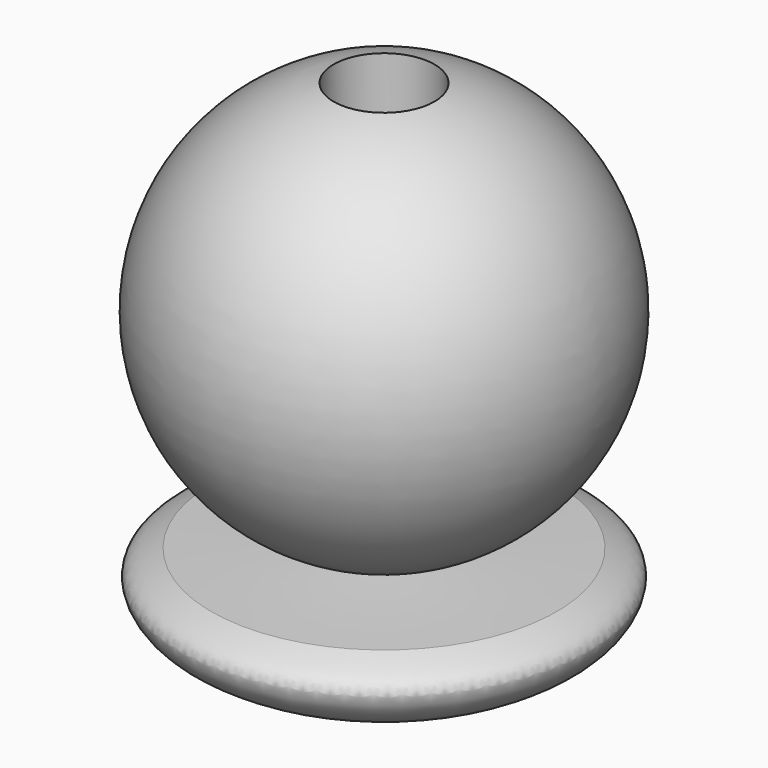
from build123d import *


with BuildPart() as f1:
    # F0 (on Front) → F1 (revolve)
    with BuildSketch(Plane.XZ):
        with BuildLine():
            Line((0, -57.654262), (0, -58.470906))
            ThreePointArc((0, -58.470906), (24.864604, -36.49857), (6.118411, -9.11952))
            Line((6.118411, -9.11952), (6.118411, -19.531853))
            Line((6.118411, -19.531853), (0, -19.531853))
            Line((0, -19.531853), (0, -57.654262))
        make_face()
        with BuildLine():
            add(Edge.make_bspline(
                [(0, -64.949296), (-7.149906, -65.588212), (-14.299812, -66.227128), (-20.638371, -66.641028)],
                knots=[0, 0, 0, 0, 0.116222, 0.116222, 0.116222, 0.116222], degree=3))
            Line((0, -64.949296), (0, -58.470906))
            ThreePointArc((0, -58.470906), (-2.391149, -58.356544), (-4.76047, -58.014501))
            add(Edge.make_bspline(
                [(-20.944773, -58.795822), (-18.825621, -58.741917), (-13.162246, -58.58282), (-7.942124, -58.246187), (-4.76047, -58.014501)],
                knots=[0.725625, 0.725625, 0.725625, 0.725625, 0.805048, 0.934865, 0.934865, 0.934865, 0.934865], degree=3))
            add(Edge.make_bspline(
                [(-20.944773, -58.795822), (-22.612293, -59.451996), (-25.692175, -60.667907), (-23.983517, -64.602899), (-21.792054, -65.957819), (-20.638371, -66.641028)],
                knots=[0, 0, 0, 0, 0.354851, 0.655531, 0.979062, 0.979062, 0.979062, 0.979062], degree=3))
        make_face()
    revolve(axis=Axis((0, 0, -2.235573), (0, 0, -1)))


solid = f1.part
